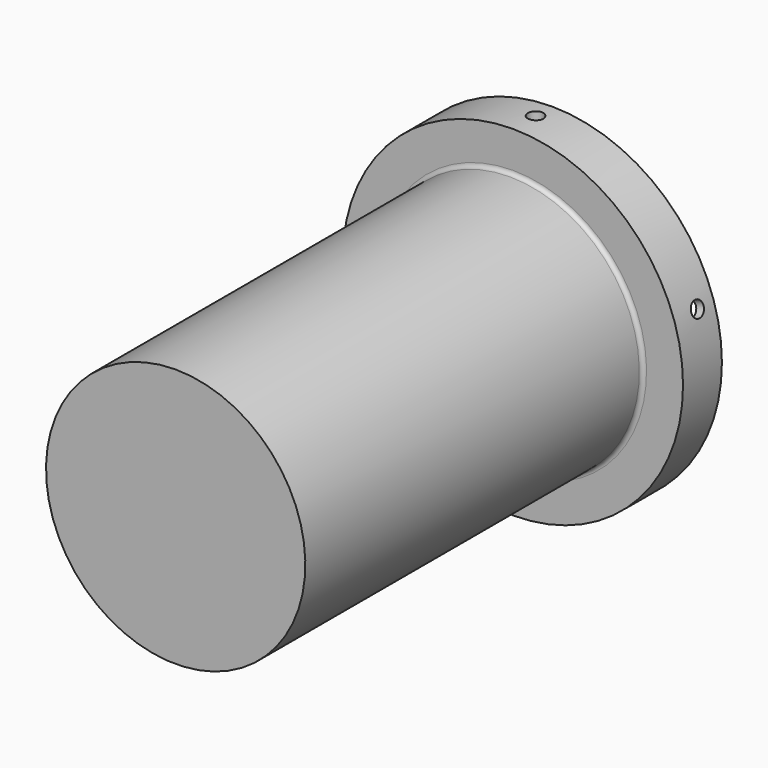
from build123d import *

# Parameters (mm, degrees)
F2_R            = 1.27
F5_D            = 4.826
F5_DEPTH        = 7.62
F5_START        = 0.0546078
F5_TIP          = 1.4498766737
F5_COPIES_COUNT = 5


# Not quite as in the source:
# - a pattern or mirror of a feature is missing from the dataset's text; its kind, count and spacing are read off the source's solid


with BuildPart() as f1:
    # F0 (on Right) → F1 (revolve)
    with BuildSketch(Plane.YZ):
        Polygon((-6.35, 50.8), (6.35, 50.8), (6.35, 53.34), (-8.89, 53.34), (-8.89, 40.64), (-135.9245181084, 40.64), (-141.0045181084, 40.64), (-141.0045181084, 0), (-135.9245181084, 0), (-135.9245181084, 38.1), (-6.35, 38.1), align=None)
    revolve(axis=Axis((0, -59.97428298, 0), (0, -1, 0)))

    # F2
    f2_edges = [f1.edges().sort_by_distance(p)[0] for p in [
        (0, -6.35, -38.1),
        (0, -6.35, -50.8),
        (0, -8.89, -40.64),
        (0, -135.924518, -38.1),
    ]]
    fillet(f2_edges, radius=F2_R)

    # F5
    # its depths count from where the whole tool has entered the part; down to there all is cleared
    with Locations(Plane.XY.offset(53.34).offset(-F5_START)):
        with Locations((0, 0)):
            f5 = Hole(F5_D / 2, depth=F5_DEPTH)
            with Locations((0, 0, -(F5_DEPTH + F5_TIP / 2))):  # 118° drill point
                Cone(0, F5_D / 2, F5_TIP, mode=Mode.SUBTRACT)

    # F5_copies: F5 ×5 about axis
    f5_copies_axis = Axis((0, 0, 0), (0, 1, 0))
    for i in range(1, F5_COPIES_COUNT):
        add(f5.rotate(f5_copies_axis, i * 360 / F5_COPIES_COUNT), mode=Mode.SUBTRACT)


solid = f1.part
